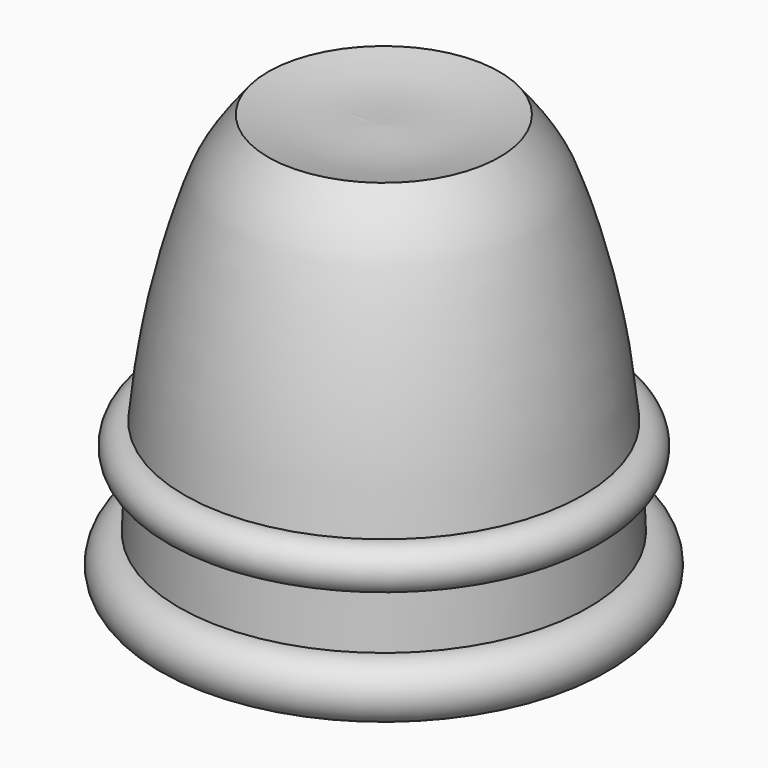
from build123d import *


# Not quite as in the source:
# - ends of sketch curves that miss each other by under 0.0002 mm in the source are joined
# - the dataset's text gives a spline's control points without its knots; the knots are read off the source's solid


with BuildPart() as f1:
    # F0 (on Front) → F1 (revolve)
    with BuildSketch(Plane.XZ):
        with BuildLine():
            add(Edge.make_bspline(
                [(0, 51.8349707127), (-2.6767978484, 51.7215871816), (-7.8655081191, 51.5018043195), (-12.4691320301, 52.5601040677), (-14.6977976302, 53.0724387607)],
                knots=[0, 0, 0, 0, 0.5158888642, 1, 1, 1, 1], degree=3))
            add(Edge.make_bspline(
                [(-14.6977976302, 53.0724387607), (-18.2147203351, 48.7739790222), (-20.1419404379, 44.4707555908), (-23.7592940633, 31.9305252816), (-25.0110844712, 22.6052167069), (-25.3571867516, 18.7494243412)],
                knots=[0, 0, 0, 0, 0.2046559912, 0.4415644707, 0.5901769055, 0.5901769055, 0.5901769055, 0.5901769055], degree=3))
            add(Edge.make_bspline(
                [(-25.3571867516, 18.7494243412), (-25.515360112, 16.9872757795), (-25.6450356494, 15.1706085799), (-25.7489504179, 13.2905869356)],
                knots=[0.5901769055, 0.5901769055, 0.5901769055, 0.5901769055, 0.6580947712, 0.6580947712, 0.6580947712, 0.6580947712], degree=3))
            add(Edge.make_bspline(
                [(-25.7489504179, 13.2905869356), (-25.8711543278, 11.0796789077), (-25.9577316296, 8.7811529991), (-26.0131338283, 6.3806387815)],
                knots=[0.6580947712, 0.6580947712, 0.6580947712, 0.6580947712, 0.7379662743, 0.7379662743, 0.7379662743, 0.7379662743], degree=3))
            add(Edge.make_bspline(
                [(-26.0131338283, 6.3806387815), (-26.0191577302, 6.1196299667), (-26.07065614, 3.7318635709), (-26.0920671828, 1.2425833051), (-26.0385365534, -0.8441913051)],
                knots=[0.7379662743, 0.7379662743, 0.7379662743, 0.7379662743, 0.7466507329, 0.8170483023, 0.8170483023, 0.8170483023, 0.8170483023], degree=3))
            Line((-26.0385365534, -0.8441913051), (-26.03099386, -0.8441206459))
            Line((-26.03099386, -0.8441206459), (-22.863238975, -0.8144454249))
            add(Edge.make_bspline(
                [(-13.2344502119, 49.8173839969), (-13.7600966459, 49.1407955568), (-14.5445414508, 48.0695229262), (-15.3630101583, 46.7891548297), (-15.9322532815, 45.7505517563), (-16.3941075068, 44.7491624028), (-16.7449950191, 43.8532384759), (-17.0306485224, 43.0558388301), (-17.2545277505, 42.4059217152), (-17.484425349, 41.720050889), (-17.9527961024, 40.2815042736), (-18.6805724441, 37.8854714001), (-19.637769837, 34.2952932796), (-20.5197777028, 30.4143486869), (-21.2563356013, 26.3660280714), (-21.8427967136, 22.1172814417), (-22.217915795, 18.3740079984), (-22.454179754, 15.2394975993), (-22.600796116, 12.813955144), (-22.718041854, 10.309340805), (-22.7923803853, 8.1521216767), (-22.8383710558, 6.382950797), (-22.8759453933, 4.5811718303), (-22.9043477549, 2.2970575919), (-22.8910974121, 0.3501033703), (-22.867178308, -0.6642488127), (-22.863238975, -0.8144454249)],
                knots=[0.021939562, 0.021939562, 0.021939562, 0.021939562, 0.0601765803, 0.0902648705, 0.1203531607, 0.1504414508, 0.180529741, 0.1955738861, 0.2106180312, 0.2256621762, 0.2407063213, 0.3008829017, 0.361059482, 0.4212360623, 0.4814126427, 0.541589223, 0.6017658033, 0.6318540935, 0.6619423837, 0.6920306738, 0.722118964, 0.7371631091, 0.7522072542, 0.7822955443, 0.8123838345, 0.8176518315, 0.8176518315, 0.8176518315, 0.8176518315], degree=3))
            Line((-13.2344502119, 49.8173839969), (0, 49.8174510092))
            Line((0, 49.8174510092), (0, 51.8349707127))
        make_face()
        with BuildLine():
            add(Edge.make_bspline(
                [(-25.3571867516, 18.7494243412), (-25.515360112, 16.9872757795), (-25.6450356494, 15.1706085799), (-25.7489504179, 13.2905869356)],
                knots=[0.5901769055, 0.5901769055, 0.5901769055, 0.5901769055, 0.6580947712, 0.6580947712, 0.6580947712, 0.6580947712], degree=3))
            ThreePointArc((-25.3571867516, 18.7494243412), (-28.3059764683, 16.2175732164), (-25.7489504179, 13.2905869356))
        make_face()
        with BuildLine():
            add(Edge.make_bspline(
                [(-26.0131338283, 6.3806387815), (-26.0191577302, 6.1196299667), (-26.07065614, 3.7318635709), (-26.0920671828, 1.2425833051), (-26.0385365534, -0.8441913051)],
                knots=[0.7379662743, 0.7379662743, 0.7379662743, 0.7379662743, 0.7466507329, 0.8170483023, 0.8170483023, 0.8170483023, 0.8170483023], degree=3))
            ThreePointArc((-26.0131338283, 6.3806387815), (-29.6812752877, 2.7810763782), (-26.0385365534, -0.8441913051))
        make_face()
    revolve(axis=Axis((0, 0, 50.8262108609), (0, 0, -1)))


solid = f1.part
